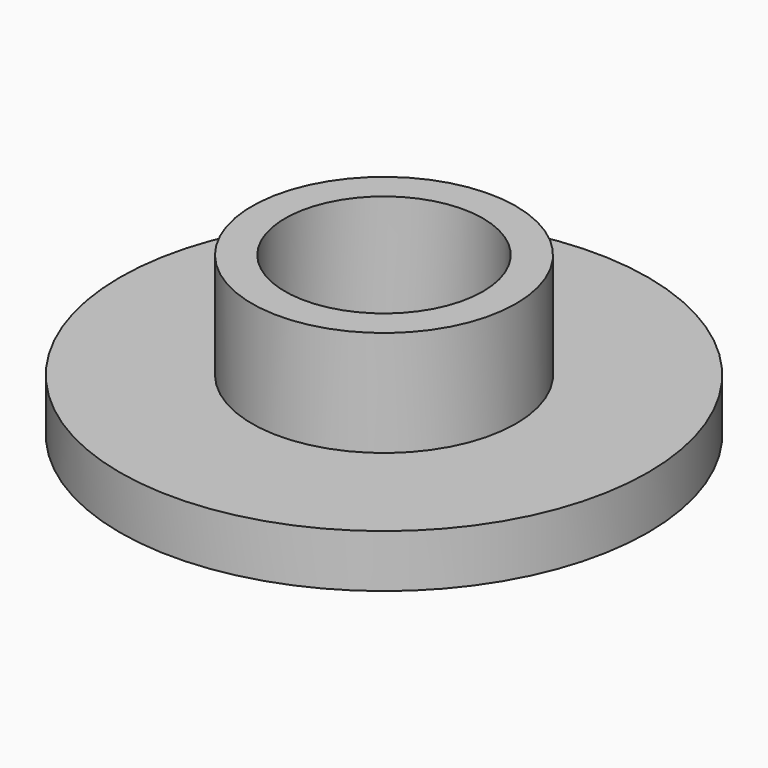
from build123d import *

# Parameters (mm, degrees)
F0_R     = 127
F0_R_2   = 47.625
F1_DEPTH = 25.4
F3_R     = 63.4843709873
F3_R_2   = 47.5995824196
F4_DEPTH = 50.8


# Not quite as in the source:
# - the program builds the solid bodies; features that only make, move or delete a surface that nothing else refers to are left out


with BuildPart() as f1:
    # F0 (on Top) → F1 (new body)
    with BuildSketch(Plane.XY):
        Circle(F0_R)
        Circle(F0_R_2, mode=Mode.SUBTRACT)
    extrude(amount=F1_DEPTH)

    # F3 (on face) → F4 (join)
    with BuildSketch(Plane.XY.offset(25.4)):
        Circle(F3_R)
        Circle(F3_R_2, mode=Mode.SUBTRACT)
    extrude(amount=F4_DEPTH)


solid = f1.part
